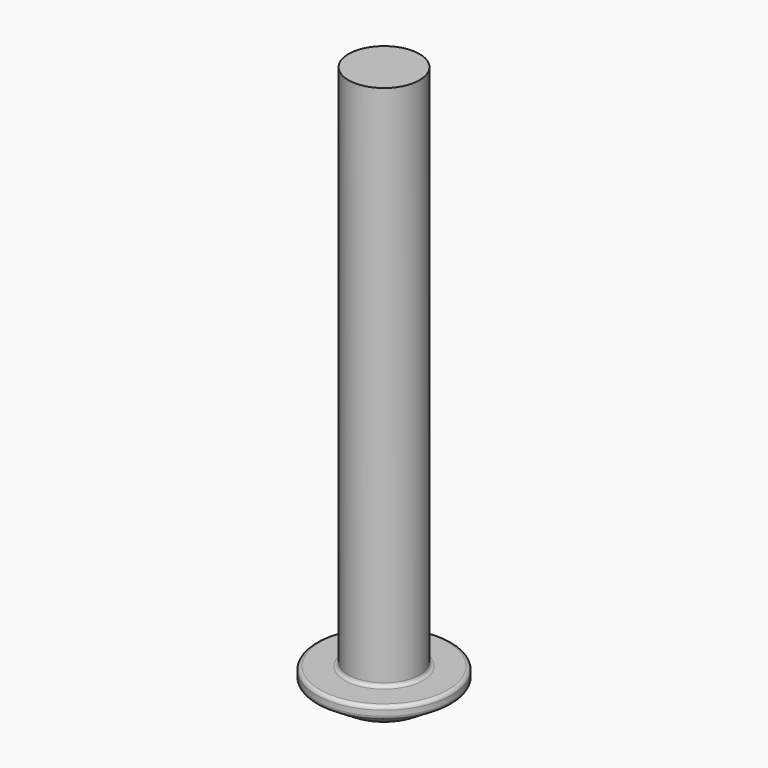
from build123d import *

# Parameters (mm, degrees)
F1_R     = 4.625
F1_R_2   = 2.425
F2_DEPTH = 2
F3_START = 1.5
F3_DEPTH = 0.5
F4_START = 2
F4_DEPTH = 36
F5_SIZE2 = 2
F5_SIZE  = 1.25
F6_R     = 0.25


# Not quite as in the source:
# - a feature names something its author has since deleted; it is built from what else it names


with BuildPart() as f2:
    # F1 (on Top) → F2 (new body)
    with BuildSketch(Plane.XY):
        Circle(F1_R)
        Circle(F1_R_2, mode=Mode.SUBTRACT)
        Circle(F1_R_2)
        Polygon((-0.9381941874, -1.625), (-1.8763883749, 0), (-0.9381941874, 1.625), (0.9381941874, 1.625), (1.8763883749, 0), (0.9381941874, -1.625), align=None, mode=Mode.SUBTRACT)
    extrude(amount=F2_DEPTH)

    # F1 (on Top) → F3 (join)
    with BuildSketch(Plane.XY.offset(F3_START)):
        Polygon((-0.9381941874, 1.625), (-1.8763883749, 0), (-0.9381941874, -1.625), (0.9381941874, -1.625), (1.8763883749, 0), (0.9381941874, 1.625), align=None)
    extrude(amount=F3_DEPTH)

    # F1 (on Top) → F4 (join)
    with BuildSketch(Plane.XY.offset(F4_START)):
        Circle(F1_R_2)
        Polygon((-0.9381941874, -1.625), (-1.8763883749, 0), (-0.9381941874, 1.625), (0.9381941874, 1.625), (1.8763883749, 0), (0.9381941874, -1.625), align=None, mode=Mode.SUBTRACT)
        Polygon((-0.9381941874, 1.625), (-1.8763883749, 0), (-0.9381941874, -1.625), (0.9381941874, -1.625), (1.8763883749, 0), (0.9381941874, 1.625), align=None)
    extrude(amount=F4_DEPTH)

    # F5
    f5_edges = [f2.edges().sort_by_distance(p)[0] for p in [
        (-4.625, 0, 0),
    ]]
    f5_side = f2.faces().sort_by_distance((-4.625, 0, 1))[0]
    chamfer(f5_edges, length=F5_SIZE, length2=F5_SIZE2, reference=f5_side)

    # F6
    f6_edges = [f2.edges().sort_by_distance(p)[0] for p in [
        (-4.625, 0, 2),
        (-2.425, 0, 2),
        (-2.625, 0, 0),
        (-4.625, 0, 1.25),
    ]]
    fillet(f6_edges, radius=F6_R)


solid = f2.part
